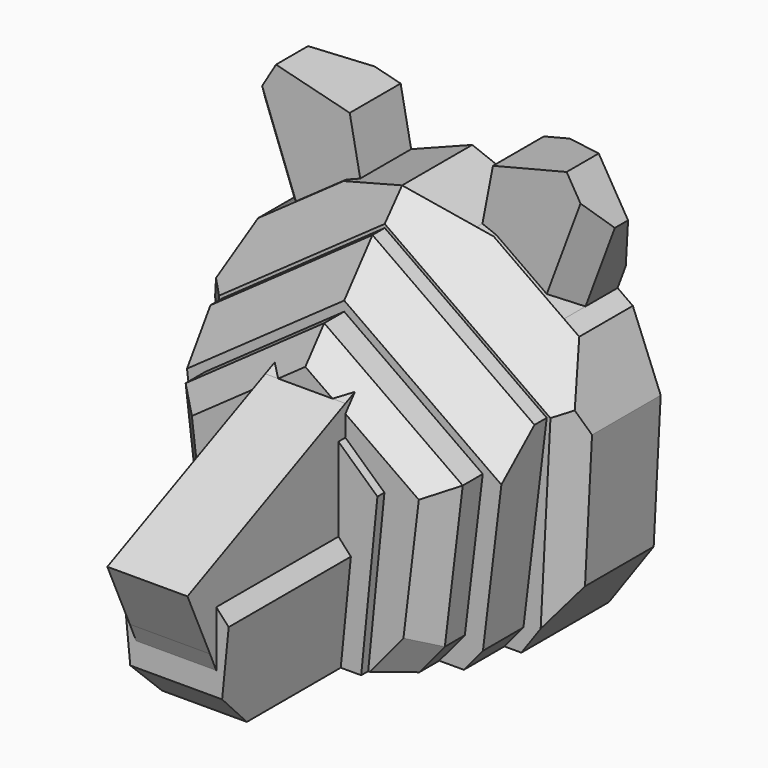
from build123d import *

# Parameters (mm, degrees)
F2_DEPTH      = 39.8739650846
F3_DEPTH      = 23.4188
F4_DEPTH      = 2.5338120759
F5_DEPTH      = 2.5338120759
F6_DEPTH      = 4.318
F7_DEPTH      = 4.318
F8_DEPTH      = 4.318
F9_DEPTH      = 4.318
F10_DEPTH     = 22.479
F11_DEPTH     = 6.858
F12_DEPTH     = 6.858
F13_SIZE      = 3.81
F14_DEPTH     = 11.7875300348
F15_T4_DEPTH  = 31.3419967727
F15_T10_DEPTH = 31.3419967727
F15_T16_DEPTH = 31.3419967727
F15_T22_DEPTH = 31.3419967727
F15_T28_DEPTH = 31.3419967727
F15_T34_DEPTH = 31.3419967727
F16_SIZE      = 2.54
F17_T1_DEPTH  = 43.0535401591
F17_T3_DEPTH  = 43.0535401591
F18_SIZE2     = 5.08
F18_SIZE      = 2.54
F19_SIZE2     = 2.54
F19_SIZE      = 5.08
F20_SIZE      = 2.54
F20_2_SIZE    = 2.54
F21_SIZE      = 2.54
F22_SIZE      = 2.54
F23_DEPTH     = 17.2466
F24_SIZE      = 3.81


# Not quite as in the source:
# - a fillet or chamfer that OpenCascade refuses, or shapes differently, is made with other operations: its cross-section is extruded or revolved along the edge and cut away or added


with BuildPart() as f2:
    # F0 (on Front) → F2 (new body, through all)
    with BuildSketch(Plane.XZ):
        Polygon((-5.6564622056, 10.8933445899), (-4.5672636413, 0), (4.5672636413, 0), (5.6564622056, 10.8933445899), (2.5338120759, 14.3030425534), (0, 14.3030425534), (-2.5338120759, 14.3030425534), align=None)
    extrude(amount=F2_DEPTH)

    # F0 (on Front) → F3 (join)
    with BuildSketch(Plane.XZ):
        Polygon((2.5338120759, 22.999221459), (0, 22.999221459), (-2.5338120759, 22.999221459), (-8.5202902555, 17.5167191774), (-6.7688368594, 0), (-4.5672636413, 0), (-5.6564622056, 10.8933445899), (-2.5338120759, 14.3030425534), (0, 14.3030425534), (2.5338120759, 14.3030425534), (5.6564622056, 10.8933445899), (4.5672636413, 0), (6.7688368594, 0), (8.5202902555, 17.5167191774), align=None)
    extrude(amount=F3_DEPTH)

    # F1 (on Right) → F4 (join, through all)
    with BuildSketch(Plane.YZ):
        Polygon((-24.4880802929, 0), (-22.7810184772, 18.4260877826), (-39.8739650846, 13.7478467077), (-40.7163016498, 8.2610081881), (-37.5194847584, 1.0165241547), align=None)
    extrude(amount=F4_DEPTH)

    # F1 (on Right) → F5 (join, through all)
    with BuildSketch(Plane.YZ):
        Polygon((-24.4880802929, 0), (-22.7810184772, 18.4260877826), (-39.8739650846, 13.7478467077), (-40.7163016498, 8.2610081881), (-37.5194847584, 1.0165241547), align=None)
    extrude(amount=-F5_DEPTH)

    # F1 (on Right) → F6 (join)
    with BuildSketch(Plane.YZ):
        Polygon((-22.7810184772, 18.4260877826), (-22.196745819, 24.7327482608), (-43.7525391617, 14.9538140945), (-40.7163016498, 8.2610081881), (-39.8739650846, 13.7478467077), align=None)
    extrude(amount=F6_DEPTH)

    # F1 (on Right) → F7 (join)
    with BuildSketch(Plane.YZ):
        Polygon((-22.7810184772, 18.4260877826), (-22.196745819, 24.7327482608), (-43.7525391617, 14.9538140945), (-40.7163016498, 8.2610081881), (-39.8739650846, 13.7478467077), align=None)
    extrude(amount=-F7_DEPTH)

    # F1 (on Right) → F8 (join)
    with BuildSketch(Plane.YZ):
        Polygon((-24.4880802929, 0), (-22.7810184772, 18.4260877826), (-39.8739650846, 13.7478467077), (-40.7163016498, 8.2610081881), (-37.5194847584, 1.0165241547), align=None)
    extrude(amount=F8_DEPTH)

    # F1 (on Right) → F9 (join)
    with BuildSketch(Plane.YZ):
        Polygon((-24.4880802929, 0), (-22.7810184772, 18.4260877826), (-39.8739650846, 13.7478467077), (-40.7163016498, 8.2610081881), (-37.5194847584, 1.0165241547), align=None)
    extrude(amount=-F9_DEPTH)

    # F0 (on Front) → F10 (join)
    with BuildSketch(Plane.XZ):
        Polygon((-2.5338120759, 22.999221459), (0, 22.999221459), (2.5338120759, 22.999221459), (8.5202902555, 17.5167191774), (6.7688368594, 0), (10.2427834645, 0), (12.9992077127, 3.318562638), (14.928705059, 19.2369148135), (0, 29.7826942206), (-14.928705059, 19.2369148135), (-12.9992077127, 3.318562638), (-10.2427834645, 0), (-6.7688368594, 0), (-8.5202902555, 17.5167191774), align=None)
    extrude(amount=F10_DEPTH)

    # F13
    f13_edges = [f2.edges().sort_by_distance(p)[0] for p in [
        (0, -39.873965, 0),
    ]]
    chamfer(f13_edges, length=F13_SIZE)

    # F15: chamfer of 2.54 on 2 edges, made by hand


with BuildPart() as f11:
    # F0 (on Front) → F11 (new body)
    with BuildSketch(Plane.XZ):
        Polygon((-18.8178192778, 38.5874472558), (-15.6579893082, 30.1085207639), (-8.0853653706, 35.4578944211), (-6.5828679126, 36.0394569064), (-7.71546131, 41.899394244), (-15.6579893082, 43.8978375339), align=None)
    extrude(amount=F11_DEPTH)

    # F18
    f18_edges = [f11.edges().sort_by_distance(p)[0] for p in [
        (-17.237904, 0, 41.242642),
    ]]
    f18_side = f11.faces().sort_by_distance((-17.237904, -3.429, 41.242642))[0]
    chamfer(f18_edges, length=F18_SIZE, length2=F18_SIZE2, reference=f18_side)

    # F20
    f20_edges = [f11.edges().sort_by_distance(p)[0] for p in [
        (-17.237904, -6.858, 34.347984),
    ]]
    chamfer(f20_edges, length=F20_SIZE)


with BuildPart() as f12:
    # F0 (on Front) → F12 (new body)
    with BuildSketch(Plane.XZ):
        Polygon((8.0853653706, 35.4578944211), (15.6579893082, 30.1085207639), (18.8178192778, 38.5874472558), (15.6579893082, 43.8978375339), (7.71546131, 41.899394244), (6.5828679126, 36.0394569064), align=None)
    extrude(amount=F12_DEPTH)

    # F19
    f19_edges = [f12.edges().sort_by_distance(p)[0] for p in [
        (17.237904, 0, 41.242642),
    ]]
    f19_side = f12.faces().sort_by_distance((12.965594, 0, 37.738789))[0]
    chamfer(f19_edges, length=F19_SIZE, length2=F19_SIZE2, reference=f19_side)

    # F20#2
    f20_2_edges = [f12.edges().sort_by_distance(p)[0] for p in [
        (17.237904, -6.858, 34.347984),
    ]]
    chamfer(f20_2_edges, length=F20_2_SIZE)


with BuildPart() as f14:
    # F0 (on Front) → F14 (new body, through all)
    with BuildSketch(Plane.XZ):
        Polygon((-14.7188181917, 0), (-12.8946364057, 0), (-14.9466200506, 2.4704601485), (-17.4552400274, 23.1665737461), (0, 35.4971215129), (17.4552400274, 23.1665737461), (14.9466200506, 2.4704601485), (12.8946364057, 0), (14.7188181917, 0), (19.5457171649, 6.8330038339), (20.3037317842, 21.4420538396), (17.3015593183, 28.9474872584), (15.6579893082, 30.1085207639), (8.0853653706, 35.4578944211), (6.5828679126, 36.0394569064), (0, 38.5874472558), (-6.5828679126, 36.0394569064), (-8.0853653706, 35.4578944211), (-15.6579893082, 30.1085207639), (-17.3015593183, 28.9474872584), (-20.3037317842, 21.4420538396), (-19.5457171649, 6.8330038339), align=None)
    extrude(amount=F14_DEPTH)

    # F17: chamfer of 4.318 x 4.572 on 2 edges, made by hand

    # F17_s2 → F17_t1 (cut)
    with BuildSketch(Plane(origin=(-7.5110021569, 0, -5.3058434446), x_dir=(0, 1, 0), z_dir=(0.816764956, 0, 0.5769705423))):
        Polygon((-11.7875300348, 29.307783219), (-7.2155300348, 33.625783219), (-11.7875300348, 33.625783219), align=None)
    extrude(amount=F17_T1_DEPTH, mode=Mode.SUBTRACT)

    # F17_s4 → F17_t3 (cut)
    with BuildSketch(Plane(origin=(-27.6536206766, 0, 19.534780968), x_dir=(0, 1, 0), z_dir=(0.816764956, 0, -0.5769705423))):
        Polygon((-11.7875300348, 29.307783219), (-7.2155300348, 33.625783219), (-11.7875300348, 33.625783219), align=None)
    extrude(amount=F17_T3_DEPTH, mode=Mode.SUBTRACT)

    # F21
    f21_edges = [f14.edges().sort_by_distance(p)[0] for p in [
        (-19.924724, -11.78753, 14.137529),
        (19.924724, -11.78753, 14.137529),
    ]]
    chamfer(f21_edges, length=F21_SIZE)


with BuildPart() as f15_tool2:
    # F15_s3 → F15_t4 (new body)
    with BuildSketch(Plane(origin=(19.3702441645, 0, 13.6833249243), x_dir=(0, 1, 0), z_dir=(-0.816764956, 0, -0.5769705423))):
        Polygon((-22.479, -21.7854609346), (-19.939, -24.3254609346), (-22.479, -24.3254609346), align=None)
    extrude(amount=F15_T4_DEPTH)

    split(bisect_by=Plane(origin=(0, -13.0936420454, 28.8624340069), x_dir=(1, 0, 0), z_dir=(0, -0.4131322018, 0.9106710624)), keep=Keep.TOP)

    split(bisect_by=Plane.YZ.offset(-4.318), keep=Keep.TOP)


with BuildPart() as f2_1:
    add(f2.part)

    # F15_t1: cut F15_tool2
    add(f15_tool2.part, mode=Mode.SUBTRACT)


with BuildPart() as f15_tool8:
    # F15_s9 → F15_t10 (new body)
    with BuildSketch(Plane(origin=(19.3702441645, 0, 13.6833249243), x_dir=(0, 1, 0), z_dir=(-0.816764956, 0, -0.5769705423))):
        Polygon((-22.479, -21.7854609346), (-19.939, -24.3254609346), (-22.479, -24.3254609346), align=None)
    extrude(amount=F15_T10_DEPTH)

    split(bisect_by=Plane(origin=(0, -13.0936420454, 28.8624340069), x_dir=(1, 0, 0), z_dir=(0, -0.4131322018, 0.9106710624)), keep=Keep.TOP)

    split(bisect_by=Plane.YZ.offset(-4.318), keep=Keep.BOTTOM)


with BuildPart() as f2_2:
    add(f2_1.part)

    # F15_t7: cut F15_tool8
    add(f15_tool8.part, mode=Mode.SUBTRACT)


with BuildPart() as f15_tool14:
    # F15_s15 → F15_t16 (new body)
    with BuildSketch(Plane(origin=(19.3702441645, 0, 13.6833249243), x_dir=(0, 1, 0), z_dir=(-0.816764956, 0, -0.5769705423))):
        Polygon((-22.479, -21.7854609346), (-19.939, -24.3254609346), (-22.479, -24.3254609346), align=None)
    extrude(amount=F15_T16_DEPTH)

    split(bisect_by=Plane(origin=(0, -13.0936420454, 28.8624340069), x_dir=(1, 0, 0), z_dir=(0, 0.4131322018, -0.9106710624)), keep=Keep.TOP)

    split(bisect_by=Plane.YZ.offset(-4.318), keep=Keep.BOTTOM)


with BuildPart() as f2_3:
    add(f2_2.part)

    # F15_t13: cut F15_tool14
    add(f15_tool14.part, mode=Mode.SUBTRACT)


with BuildPart() as f15_tool20:
    # F15_s21 → F15_t22 (new body)
    with BuildSketch(Plane(origin=(6.2288004504, 0, -4.4000839497), x_dir=(0, 1, 0), z_dir=(-0.816764956, 0, 0.5769705423))):
        Polygon((-22.479, -21.7854609346), (-19.939, -24.3254609346), (-22.479, -24.3254609346), align=None)
    extrude(amount=F15_T22_DEPTH)

    split(bisect_by=Plane.YZ.offset(4.318), keep=Keep.TOP)

    split(bisect_by=Plane(origin=(0, -13.0936420454, 28.8624340069), x_dir=(1, 0, 0), z_dir=(0, 0.4131322018, -0.9106710624)), keep=Keep.TOP)


with BuildPart() as f2_4:
    add(f2_3.part)

    # F15_t19: cut F15_tool20
    add(f15_tool20.part, mode=Mode.SUBTRACT)


with BuildPart() as f15_tool26:
    # F15_s27 → F15_t28 (new body)
    with BuildSketch(Plane(origin=(6.2288004504, 0, -4.4000839497), x_dir=(0, 1, 0), z_dir=(-0.816764956, 0, 0.5769705423))):
        Polygon((-22.479, -21.7854609346), (-19.939, -24.3254609346), (-22.479, -24.3254609346), align=None)
    extrude(amount=F15_T28_DEPTH)

    split(bisect_by=Plane.YZ.offset(4.318), keep=Keep.TOP)

    split(bisect_by=Plane(origin=(0, -13.0936420454, 28.8624340069), x_dir=(1, 0, 0), z_dir=(0, -0.4131322018, 0.9106710624)), keep=Keep.TOP)


with BuildPart() as f2_5:
    add(f2_4.part)

    # F15_t25: cut F15_tool26
    add(f15_tool26.part, mode=Mode.SUBTRACT)


with BuildPart() as f15_tool32:
    # F15_s33 → F15_t34 (new body)
    with BuildSketch(Plane(origin=(6.2288004504, 0, -4.4000839497), x_dir=(0, 1, 0), z_dir=(-0.816764956, 0, 0.5769705423))):
        Polygon((-22.479, -21.7854609346), (-19.939, -24.3254609346), (-22.479, -24.3254609346), align=None)
    extrude(amount=F15_T34_DEPTH)

    split(bisect_by=Plane.YZ.offset(4.318), keep=Keep.BOTTOM)

    split(bisect_by=Plane(origin=(0, -13.0936420454, 28.8624340069), x_dir=(1, 0, 0), z_dir=(0, -0.4131322018, 0.9106710624)), keep=Keep.TOP)


with BuildPart() as f2_6:
    add(f2_5.part)

    # F15_t31: cut F15_tool32
    add(f15_tool32.part, mode=Mode.SUBTRACT)

    # F16
    f16_edges = [f2_6.edges().sort_by_distance(p)[0] for p in [
        (-11.620996, -22.479, 1.659281),
        (11.620996, -22.479, 1.659281),
    ]]
    chamfer(f16_edges, length=F16_SIZE)

    # F22
    f22_edges = [f2_6.edges().sort_by_distance(p)[0] for p in [
        (-14.072441, -22.479, 12.172733),
        (14.072441, -22.479, 12.172733),
    ]]
    chamfer(f22_edges, length=F22_SIZE)


with BuildPart() as f23:
    # F0 (on Front) → F23 (new body)
    with BuildSketch(Plane.XZ):
        Polygon((-12.8946364057, 0), (-10.2427834645, 0), (-12.9992077127, 3.318562638), (-14.928705059, 19.2369148135), (0, 29.7826942206), (14.928705059, 19.2369148135), (12.9992077127, 3.318562638), (10.2427834645, 0), (12.8946364057, 0), (14.9466200506, 2.4704601485), (17.4552400274, 23.1665737461), (0, 35.4971215129), (-17.4552400274, 23.1665737461), (-14.9466200506, 2.4704601485), align=None)
    extrude(amount=F23_DEPTH)

    # F24
    f24_edges = [f23.edges().sort_by_distance(p)[0] for p in [
        (-8.72762, -17.2466, 29.331848),
        (8.72762, -17.2466, 29.331848),
    ]]
    chamfer(f24_edges, length=F24_SIZE)


solid = Compound([f11.part, f12.part, f14.part, f2_6.part, f23.part])
